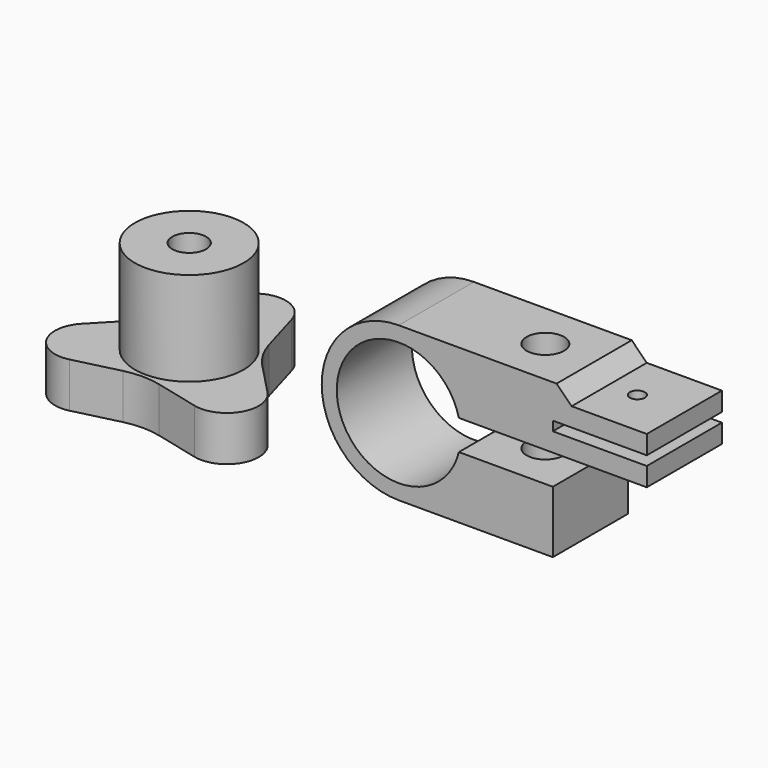
from build123d import *

# Parameters (mm, degrees)
F0_R        = 14.4655577075
F0_W        = 10.5
F0_H        = 10.5
F1_DEPTH    = 12
F0_R_2      = 4.5
F2_DEPTH    = 25
F3_R        = 10
F3_W        = 10.5
F3_H        = 10.5
F4_DEPTH    = 5
F6_DEPTH    = 25
F7_W        = 25
F7_H        = 5
F8_DEPTH    = 25
F9_T4_DEPTH = 25
F10_R       = 5
F10_R_2     = 2
F11_DEPTH   = 41.001


# Not quite as in the source:
# - a fillet or chamfer that OpenCascade refuses, or shapes differently, is made with other operations: its cross-section is extruded or revolved along the edge and cut away or added


with BuildPart() as f1:
    # F0 (on Top) → F1 (new body)
    with BuildSketch(Plane.XY):
        with BuildLine():
            Line((11.5311605337, 12.1863566004), (8.1457248267, 23.8782938791))
            ThreePointArc((8.1457248267, 23.8782938791), (0, 30), (-8.1457248267, 23.8782938791))
            Line((-8.1457248267, 23.8782938791), (-11.5311605337, 12.1863566004))
            ThreePointArc((-11.5311605337, 12.1863566004), (-13.4215306345, 7.7489243248), (-16.3192746623, 3.8930996571))
            Line((-16.3192746623, 3.8930996571), (-24.7520715117, -4.8847423074))
            ThreePointArc((-24.7520715117, -4.8847423074), (-25.9807621135, -15), (-16.606346685, -18.9935515717))
            Line((-16.606346685, -18.9935515717), (-4.7881141286, -16.0794562575))
            ThreePointArc((-4.7881141286, -16.0794562575), (0, -15.4978486495), (4.7881141286, -16.0794562575))
            Line((4.7881141286, -16.0794562575), (16.606346685, -18.9935515717))
            ThreePointArc((16.606346685, -18.9935515717), (25.9807621135, -15), (24.7520715117, -4.8847423074))
            Line((24.7520715117, -4.8847423074), (16.3192746623, 3.8930996571))
            ThreePointArc((16.3192746623, 3.8930996571), (13.4215306345, 7.7489243248), (11.5311605337, 12.1863566004))
        make_face()
        Circle(F0_R, mode=Mode.SUBTRACT)
        Circle(F0_R)
        Rectangle(F0_W, F0_H, mode=Mode.SUBTRACT)
    extrude(amount=-F1_DEPTH)

    # F0 (on Top) → F2 (join)
    with BuildSketch(Plane.XY):
        Circle(F0_R)
        Rectangle(F0_W, F0_H, mode=Mode.SUBTRACT)
        Rectangle(F0_W, F0_H)
        Circle(F0_R_2, mode=Mode.SUBTRACT)
    extrude(amount=F2_DEPTH)

    # F3 (on face) → F4 (cut)
    with BuildSketch(Plane(origin=(0, 0, -12), x_dir=(1, 0, 0), z_dir=(0, 0, -1))):
        Circle(F3_R)
        Rectangle(F3_W, F3_H, mode=Mode.SUBTRACT)
    extrude(amount=-F4_DEPTH, mode=Mode.SUBTRACT)


with BuildPart() as f6:
    # F5 (on Front) → F6 (new body)
    with BuildSketch(Plane.XZ):
        with BuildLine():
            ThreePointArc((91.7727594808, 16.0042379603), (59.2649488872, 20.0042379603), (91.7727594808, 24.0042379603))
            Line((91.7727594808, 24.0042379603), (116.7727594808, 24.0042379603))
            Line((116.7727594808, 24.0042379603), (116.7727594808, 40.5042379603))
            Line((116.7727594808, 40.5042379603), (75.7649488872, 40.5042379603))
            ThreePointArc((75.7649488872, 40.5042379603), (55.2649488872, 20.0042379603), (75.7649488872, -0.4957620397))
            Line((75.7649488872, -0.4957620397), (116.7727594808, -0.4957620397))
            Line((116.7727594808, -0.4957620397), (116.7727594808, 16.0042379603))
            Line((116.7727594808, 16.0042379603), (91.7727594808, 16.0042379603))
        make_face()
    extrude(amount=F6_DEPTH)

    # F7 (on face) → F8 (join)
    with BuildSketch(Plane.YZ.offset(116.7727594808)):
        with Locations((-12.5, 26.5042379603)):
            Rectangle(F7_W, F7_H)
        with Locations((-12.5, 34.0042379603)):
            Rectangle(F7_W, F7_H)
    extrude(amount=F8_DEPTH)

    # F9: chamfer of 5 on 1 edges, made by hand


with BuildPart() as f9_tool2:
    # F9_s3 → F9_t4 (new body)
    with BuildSketch(Plane.XZ):
        Polygon((116.7727594808, 41.5042379603), (121.7727594808, 36.5042379603), (116.7727594808, 36.5042379603), align=None)
    extrude(amount=F9_T4_DEPTH)

    split(bisect_by=Plane.XY.offset(40.5042379603), keep=Keep.BOTTOM)


with BuildPart() as f6_1:
    add(f6.part)

    # F9_t1: union F9_tool2
    add(f9_tool2.part)

    # F10 (on face) → F11 (cut, through all)
    with BuildSketch(Plane(origin=(0, 0, -0.4957620397), x_dir=(1, 0, 0), z_dir=(0, 0, -1))):
        with Locations((104.7727594808, 12.5)):
            Circle(F10_R)
        with Locations((129.2727594808, 12.5)):
            Circle(F10_R_2)
    extrude(amount=-F11_DEPTH, mode=Mode.SUBTRACT)


solid = Compound([f1.part, f6_1.part])
